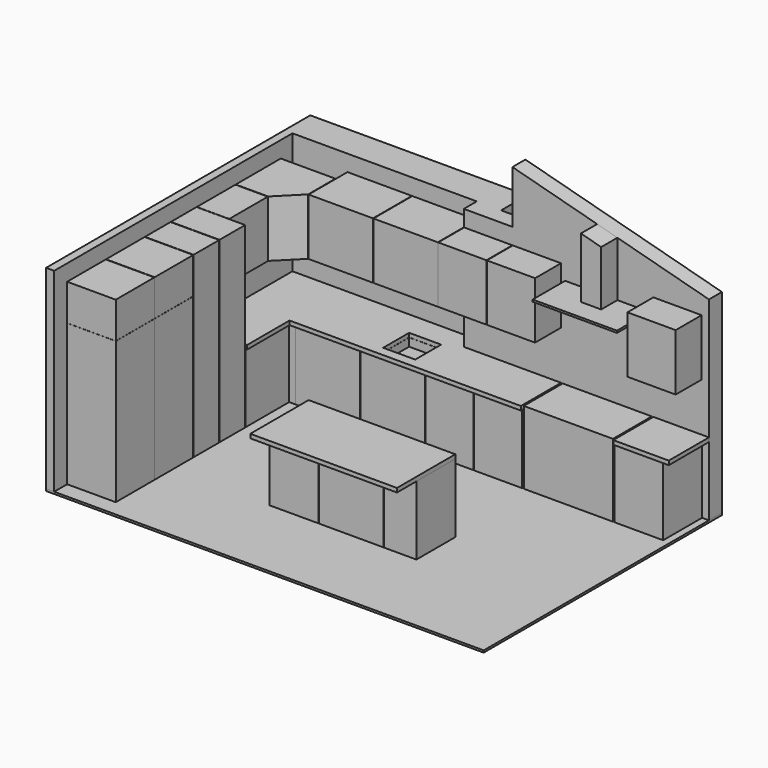
from build123d import *

# Parameters (mm, degrees)
F1_DEPTH  = 2400
F3_DEPTH  = 850
F4_W      = 600
F4_H      = 395
F5_DEPTH  = 2200
F6_DEPTH  = 2200
F4_H_2    = 595
F7_DEPTH  = 1750
F8_DEPTH  = 1750
F2_W      = 795
F2_H      = 600
F9_DEPTH  = 850
F10_DEPTH = 850
F2_W_2    = 595
F11_DEPTH = 850
F12_DEPTH = 850
F2_W_3    = 1100
F13_DEPTH = 900
F2_W_4    = 600
F14_DEPTH = 850
F16_W     = 795
F16_H     = 600
F17_DEPTH = 700
F18_DEPTH = 700
F19_DEPTH = 25
F16_W_2   = 595
F16_H_2   = 400
F20_DEPTH = 700
F22_DEPTH = 200
F24_DEPTH = 250
F25_DEPTH = 500
F26_DEPTH = 700
F16_W_3   = 400
F16_H_3   = 595
F27_DEPTH = 700
F31_DEPTH = 50
F30_W     = 685
F30_H     = 620
F28_W     = 395
F28_H     = 400
F32_DEPTH = 100
F33_W     = 600
F33_H     = 595
F34_DEPTH = 449
F35_W     = 600
F35_H     = 600
F36_DEPTH = 850
F35_W_2   = 800
F35_W_3   = 400
F37_W     = 600
F37_H     = 600
F38_DEPTH = 50


# Not quite as in the source:
# - a feature names something its author has since deleted; it is built from what else it names


with BuildPart() as f1:
    # F0 (on Top) → F1 (new body)
    with BuildSketch(Plane.XY):
        Polygon((0, -3475), (0, 200), (2275, 200), (2275, 0), (5300, 0), (5300, 200), (2575, 200), (2575, 600), (-100, 600), (-100, -3475), align=None)
    extrude(amount=F1_DEPTH)

    # F21 (on face) → F22 (join)
    with BuildSketch(Plane.XZ):
        Polygon((2875, 2400), (5300, 2400), (2875, 3049.7767916455), align=None)
    extrude(amount=-F22_DEPTH)


with BuildPart() as f3:
    # F2 (on Top) → F3 (new body)
    with BuildSketch(Plane.XY):
        Polygon((675, 0), (0, 0), (0, -1275), (600, -1275), (600, -600), (675, -600), align=None)
    extrude(amount=F3_DEPTH)


with BuildPart() as f5:
    # F4 (on Top) → F5 (new body)
    with BuildSketch(Plane.XY):
        with Locations((300, -1477.5)):
            Rectangle(F4_W, F4_H)
    extrude(amount=F5_DEPTH)


with BuildPart() as f6:
    # F4 (on Top) → F6 (new body)
    with BuildSketch(Plane.XY):
        with Locations((300, -1877.5)):
            Rectangle(F4_W, F4_H)
    extrude(amount=F6_DEPTH)


with BuildPart() as f7:
    # F4 (on Top) → F7 (new body)
    with BuildSketch(Plane.XY):
        with Locations((300, -2377.5)):
            Rectangle(F4_W, F4_H_2)
    extrude(amount=F7_DEPTH)


with BuildPart() as f8:
    # F4 (on Top) → F8 (new body)
    with BuildSketch(Plane.XY):
        with Locations((300, -2977.5)):
            Rectangle(F4_W, F4_H_2)
    extrude(amount=F8_DEPTH)


with BuildPart() as f9:
    # F2 (on Top) → F9 (new body)
    with BuildSketch(Plane.XY):
        with Locations((1077.5, -300)):
            Rectangle(F2_W, F2_H)
    extrude(amount=F9_DEPTH)


with BuildPart() as f10:
    # F2 (on Top) → F10 (new body)
    with BuildSketch(Plane.XY):
        with Locations((1877.5, -300)):
            Rectangle(F2_W, F2_H)
    extrude(amount=F10_DEPTH)


with BuildPart() as f11:
    # F2 (on Top) → F11 (new body)
    with BuildSketch(Plane.XY):
        with Locations((2577.5, -300)):
            Rectangle(F2_W_2, F2_H)
    extrude(amount=F11_DEPTH)


with BuildPart() as f12:
    # F2 (on Top) → F12 (new body)
    with BuildSketch(Plane.XY):
        with Locations((3177.5, -300)):
            Rectangle(F2_W_2, F2_H)
    extrude(amount=F12_DEPTH)


with BuildPart() as f13:
    # F2 (on Top) → F13 (new body)
    with BuildSketch(Plane.XY):
        with Locations((4045, -300)):
            Rectangle(F2_W_3, F2_H)
    extrude(amount=F13_DEPTH)


with BuildPart() as f14:
    # F2 (on Top) → F14 (new body)
    with BuildSketch(Plane.XY):
        with Locations((4915, -300)):
            Rectangle(F2_W_4, F2_H)
    extrude(amount=F14_DEPTH)


with BuildPart() as f17:
    # F16 (on offset) → F17 (new body)
    with BuildSketch(Plane.XY.offset(1500)):
        with Locations((1077.5, -101)):
            Rectangle(F16_W, F16_H)
    extrude(amount=F17_DEPTH)


with BuildPart() as f18:
    # F16 (on offset) → F18 (new body)
    with BuildSketch(Plane.XY.offset(1500)):
        with Locations((1877.5, -101)):
            Rectangle(F16_W, F16_H)
    extrude(amount=F18_DEPTH)


with BuildPart() as f19:
    # F0 (on Top) → F19 (new body)
    with BuildSketch(Plane.XY):
        Polygon((0, -3475), (0, 200), (2275, 200), (2275, 0), (5300, 0), (5300, 200), (2575, 200), (2575, 600), (-100, 600), (-100, -3475), align=None)
        Polygon((2275, 200), (0, 200), (0, -3475), (5300, -3475), (5300, 0), (2275, 0), align=None)
    extrude(amount=-F19_DEPTH)


with BuildPart() as f20:
    # F16 (on offset) → F20 (new body)
    with BuildSketch(Plane.XY.offset(1500)):
        with Locations((2577.5, -201)):
            Rectangle(F16_W_2, F16_H_2)
    extrude(amount=F20_DEPTH)


with BuildPart() as f20b:
    # F16 (on offset) → F20, piece 2 (new body)
    with BuildSketch(Plane.XY.offset(1500)):
        with Locations((3177.5, -201)):
            Rectangle(F16_W_2, F16_H_2)
    extrude(amount=F20_DEPTH)


with BuildPart() as f20c:
    # F16 (on offset) → F20, piece 3 (new body)
    with BuildSketch(Plane.XY.offset(1500)):
        with Locations((4912.5, -201)):
            Rectangle(F16_W_2, F16_H_2)
    extrude(amount=F20_DEPTH)


with BuildPart() as f24:
    # F23 (on face) → F24 (new body)
    with BuildSketch(Plane.XZ):
        Polygon((3920, 2769.769885555), (3920, 2025), (4170, 2025), (4170, 2702.7825874472), align=None)
    extrude(amount=F24_DEPTH)


with BuildPart() as f25:
    # F23 (on face) → F25 (new body)
    with BuildSketch(Plane.XZ):
        Polygon((3525, 2025), (3525, 2000), (4565, 2000), (4565, 2025), (4170, 2025), (3920, 2025), align=None)
    extrude(amount=F25_DEPTH)


with BuildPart() as f26:
    # F16 (on offset) → F26 (new body)
    with BuildSketch(Plane.XY.offset(1500)):
        Polygon((675, 18.8704896718), (1, 18.8704896718), (1, -676), (401, -676), (675, -401), align=None)
    extrude(amount=F26_DEPTH)


with BuildPart() as f27:
    # F16 (on offset) → F27 (new body)
    with BuildSketch(Plane.XY.offset(1500)):
        with Locations((201, -978.5)):
            Rectangle(F16_W_3, F16_H_3)
    extrude(amount=F27_DEPTH)


with BuildPart() as f31:
    # F30 (on offset) → F31 (new body)
    with BuildSketch(Plane.XY.offset(851)):
        Polygon((2275, 200), (0, 200), (0, -1274), (620, -1274), (620, -620), (3475, -620), (3475, 0), (2275, 0), align=None)
    extrude(amount=F31_DEPTH)


with BuildPart() as f31b:
    # F30 (on offset) → F31, piece 2 (new body)
    with BuildSketch(Plane.XY.offset(851)):
        with Locations((4957.5, -310)):
            Rectangle(F30_W, F30_H)
    extrude(amount=F31_DEPTH)


with BuildPart() as f32_tool:
    # F28 (on face) → F32 (new body, symmetric)
    with BuildSketch(Plane.XY.offset(850)):
        with Locations((1877.5, -300)):
            Rectangle(F28_W, F28_H)
    extrude(amount=F32_DEPTH, both=True)


with BuildPart() as f10_1:
    add(f10.part)

    # F32: cut by f32_tool
    add(f32_tool.part, mode=Mode.SUBTRACT)


with BuildPart() as f31_1:
    add(f31.part)

    # F32: cut by f32_tool
    add(f32_tool.part, mode=Mode.SUBTRACT)


with BuildPart() as f34:
    # F33 (on face) → F34 (new body)
    with BuildSketch(Plane.XY.offset(2200)):
        with Locations((300, -2977.5)):
            Rectangle(F33_W, F33_H)
    extrude(amount=-F34_DEPTH)


with BuildPart() as f34b:
    # F33 (on face) → F34, piece 2 (new body)
    with BuildSketch(Plane.XY.offset(2200)):
        with Locations((300, -2377.5)):
            Rectangle(F33_W, F33_H)
    extrude(amount=-F34_DEPTH)


with BuildPart() as f36:
    # F35 (on face) → F36 (new body)
    with BuildSketch(Plane.XY):
        with Locations((2100, -2100)):
            Rectangle(F35_W, F35_H)
    extrude(amount=F36_DEPTH)


with BuildPart() as f36b:
    # F35 (on face) → F36, piece 2 (new body)
    with BuildSketch(Plane.XY):
        with Locations((2805, -2100)):
            Rectangle(F35_W_2, F35_H)
    extrude(amount=F36_DEPTH)


with BuildPart() as f36c:
    # F35 (on face) → F36, piece 3 (new body)
    with BuildSketch(Plane.XY):
        with Locations((3410, -2100)):
            Rectangle(F35_W_3, F35_H)
    extrude(amount=F36_DEPTH)


with BuildPart() as f38:
    # F37 (on face) → F38 (new body)
    with BuildSketch(Plane.XY.offset(850)):
        Polygon((3610, -1800), (2400, -1800), (2400, -2400), (1800, -2400), (1800, -2700), (3610, -2700), align=None)
        with Locations((2100, -2100)):
            Rectangle(F37_W, F37_H)
    extrude(amount=F38_DEPTH)


solid = Compound([f1.part, f3.part, f5.part, f6.part, f7.part, f8.part, f9.part, f11.part, f12.part, f13.part, f14.part, f17.part, f18.part, f19.part, f20.part, f20b.part, f20c.part, f24.part, f25.part, f26.part, f27.part, f31b.part, f10_1.part, f31_1.part, f34.part, f34b.part, f36.part, f36b.part, f36c.part, f38.part])
